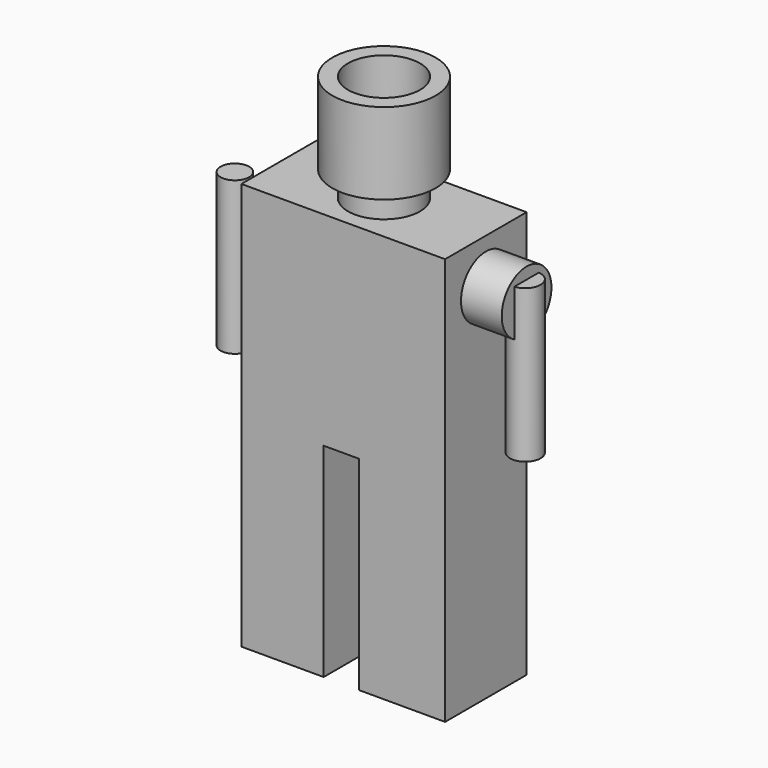
from build123d import *

# Parameters (mm, degrees)
F0_W      = 12.7
F0_H      = 6.3499995352
F1_DEPTH  = 12.7
F2_R      = 4.4917075471
F3_DEPTH  = 3.175
F4_R      = 6.4364972291
F4_R_2    = 4.4917075471
F5_DEPTH  = 10.16
F8_R      = 3.8726977567
F9_DEPTH  = 5.08
F10_W     = 10.2532109383
F10_H     = 12.6999990704
F10_W_2   = 10.7425687972
F11_DEPTH = 25.4
F12_R     = 1.7812892701
F13_DEPTH = 9.525
F12_R_2   = 1.9110034549


# Not quite as in the source:
# - the program builds the solid bodies; features that only make, move or delete a surface that nothing else refers to are left out


with BuildPart() as f1:
    # F0 (on Top) → F1 (new body, symmetric)
    with BuildSketch(Plane.XY):
        with Locations((-6.35, -3.1749997676)):
            Rectangle(F0_W, F0_H)
        with Locations((6.35, -3.1749997676)):
            Rectangle(F0_W, F0_H)
        with Locations((-6.35, 3.1749997676)):
            Rectangle(F0_W, F0_H)
        with Locations((6.35, 3.1749997676)):
            Rectangle(F0_W, F0_H)
    extrude(amount=F1_DEPTH, both=True)

    # F2 (on face) → F3 (join, symmetric)
    with BuildSketch(Plane.XY.offset(12.7)):
        Circle(F2_R)
    extrude(amount=F3_DEPTH, both=True)

    # F8 (on face) → F9 (join)
    with BuildSketch(Plane.YZ.offset(12.7)):
        with Locations((0, 7.0956880227)):
            Circle(F8_R)
    extrude(amount=F9_DEPTH)

    # F10 (on face) → F11 (join)
    with BuildSketch(Plane(origin=(0, 0, -12.7), x_dir=(1, 0, 0), z_dir=(0, 0, -1))):
        with Locations((-7.5733945308, 0)):
            Rectangle(F10_W, F10_H)
        with Locations((7.3287156014, 0)):
            Rectangle(F10_W_2, F10_H)
    extrude(amount=F11_DEPTH)


with BuildPart() as f5:
    # F4 (on face) → F5 (new body)
    with BuildSketch(Plane.XY.offset(15.875)):
        Circle(F4_R)
        Circle(F4_R_2, mode=Mode.SUBTRACT)
    extrude(amount=F5_DEPTH)


with BuildPart() as f13:
    # F12 (on Top) → F13 (new body, symmetric)
    with BuildSketch(Plane.XY):
        with Locations((-18.5955967754, 0)):
            Circle(F12_R)
    extrude(amount=F13_DEPTH, both=True)


with BuildPart() as f13b:
    # F12 (on Top) → F13, piece 2 (new body, symmetric)
    with BuildSketch(Plane.XY):
        with Locations((17.616879195, 0)):
            Circle(F12_R_2)
    extrude(amount=F13_DEPTH, both=True)


solid = Compound([f1.part, f5.part, f13.part, f13b.part])
